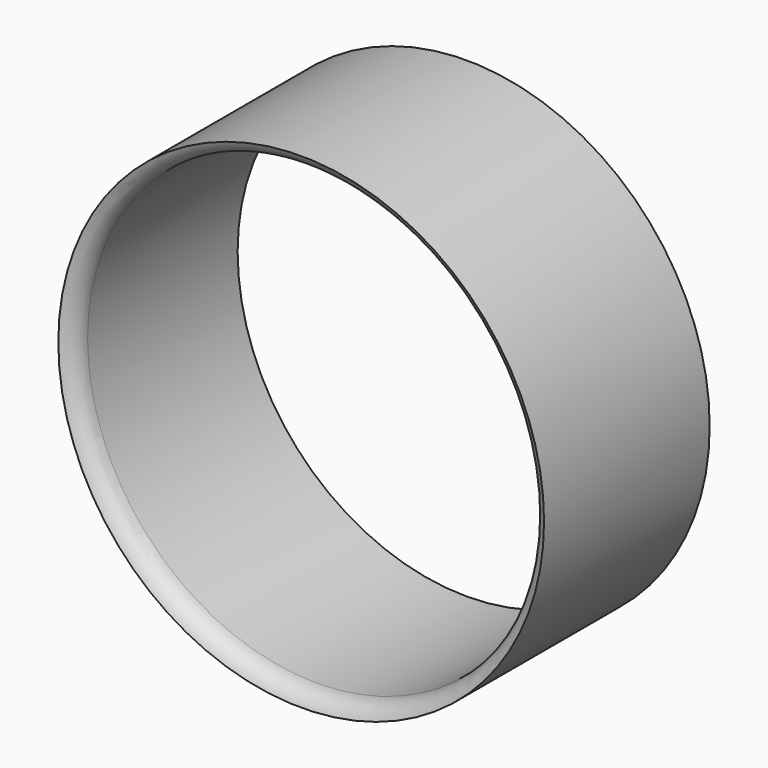
from build123d import *

# Parameters (mm, degrees)
F0_R     = 59.590133007
F0_R_2   = 56.2308790167
F1_DEPTH = 50.8


# Not quite as in the source:
# - a fillet or chamfer that OpenCascade refuses, or shapes differently, is made with other operations: its cross-section is extruded or revolved along the edge and cut away or added


with BuildPart() as f1:
    # F0 (on Front) → F1 (new body)
    with BuildSketch(Plane.XZ):
        Circle(F0_R)
        Circle(F0_R_2, mode=Mode.SUBTRACT)
    extrude(amount=F1_DEPTH)

    # F2: fillet of radius 5.08 on 1 edges, made by hand

    # F2_s1 → F2_t2 (revolve, cut)
    with BuildSketch(Plane.XY):
        with BuildLine():
            ThreePointArc((56.2308790167, -46.0203103479), (57.154691477, -48.9413555608), (59.590133007, -50.8))
            Line((59.590133007, -50.8), (56.2308790167, -50.8))
            Line((56.2308790167, -50.8), (56.2308790167, -46.0203103479))
        make_face()
    revolve(axis=Axis((0, -50.8, 0), (0, -1, 0)), mode=Mode.SUBTRACT)


solid = f1.part
